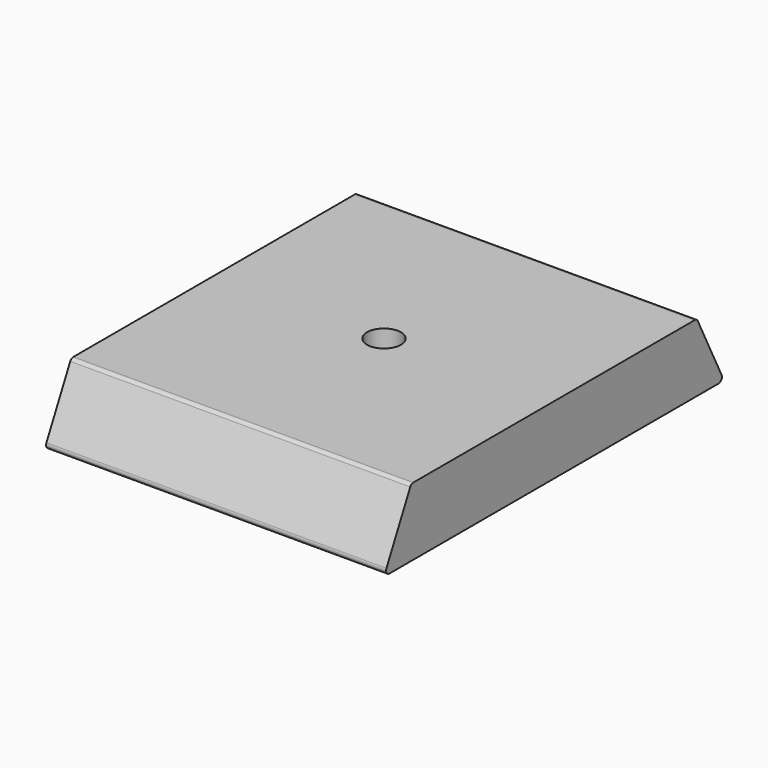
from build123d import *

# Parameters (mm, degrees)
F1_DEPTH = 40
F2_R     = 0.5
F3_T     = 4
F4_R     = 2
F5_DEPTH = 4


# Not quite as in the source:
# - a shell that OpenCascade refuses in one call is made with other operations: the cavity is built on its own and cut out


with BuildPart() as f1:
    # F0 (on Right) → F1 (new body)
    with BuildSketch(Plane.YZ):
        Polygon((4, 8), (0, 0), (50, 0), (46, 8), align=None)
    extrude(amount=F1_DEPTH)

    # F2
    f2_edges = [f1.edges().sort_by_distance(p)[0] for p in [
        (20, 4, 8),
        (20, 46, 8),
        (20, 0, 0),
        (20, 50, 0),
    ]]
    fillet(f2_edges, radius=F2_R)

    # F3: shell of thickness 4, made by hand


with BuildPart() as f3_core1:
    # F3_t2: copy of F1
    add(f1.part)

    # the walls: a layer under each face that stays
    f3_faces = [f3_core1.faces().sort_by_distance(p)[0] for p in [
        (20, 2.1118033989, 4.2236067977),
        (0, 25, 4),
        (40, 25, 4),
        (20, 25, 8),
        (20, 47.8881966011, 4.2236067977),
    ]]
    thicken(f3_faces, amount=-F3_T, mode=Mode.SUBTRACT)


with BuildPart() as f1_1:
    add(f1.part)

    # what is left inside the walls is the cavity
    f3_cavity = [f3_core1.part.solids().sort_by_distance(p)[0] for p in [
        (25.333333, 25, 0.04),
    ]]
    add(f3_cavity, mode=Mode.SUBTRACT)

    # F4 (on face) → F5 (cut, through all)
    with BuildSketch(Plane(origin=(0, 0, 4), x_dir=(1, 0, 0), z_dir=(0, 0, -1))):
        with Locations((20, -25)):
            Circle(F4_R)
    extrude(amount=-F5_DEPTH, mode=Mode.SUBTRACT)


solid = f1_1.part
